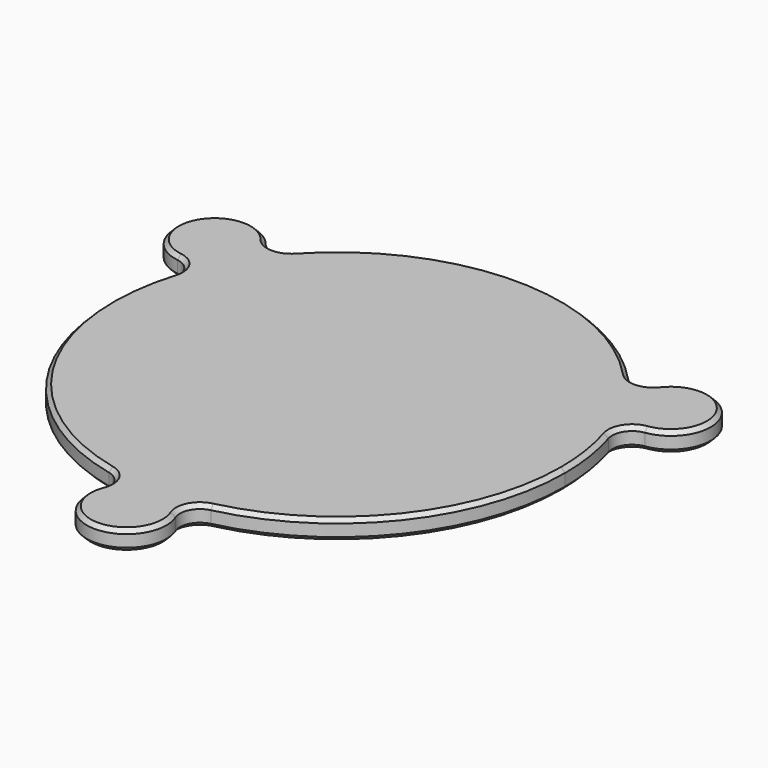
from build123d import *

# Parameters (mm, degrees)
F1_DEPTH = 5
F2_R     = 5
F3_SIZE  = 1


with BuildPart() as f1:
    # F0 (on Top) → F1 (new body)
    with BuildSketch(Plane.XY):
        with BuildLine():
            ThreePointArc((-4.0489926269, -57.0063869992), (0, -76.15), (4.0489926269, -57.0063869992))
            ThreePointArc((4.0489926269, -57.0063869992), (0, -57.15), (-4.0489926269, -57.0063869992))
        make_face()
        with BuildLine():
            ThreePointArc((4.0489926269, -57.0063869992), (41.8181923846, -38.9533218826), (57.15, 0))
            ThreePointArc((57.15, 0), (55.6922778867, 12.8254701198), (51.3934756327, 24.996663025))
            ThreePointArc((51.3934756327, 24.996663025), (49.4933518263, 28.575), (47.3444830059, 32.0097239742))
            ThreePointArc((47.3444830059, 32.0097239742), (0, 57.15), (-47.3444830059, 32.0097239742))
            ThreePointArc((-47.3444830059, 32.0097239742), (-49.4933518263, 28.575), (-51.3934756327, 24.996663025))
            ThreePointArc((-51.3934756327, 24.996663025), (-49.4933518263, -28.575), (-4.0489926269, -57.0063869992))
            ThreePointArc((-4.0489926269, -57.0063869992), (0, -57.15), (4.0489926269, -57.0063869992))
        make_face()
        with BuildLine():
            ThreePointArc((-51.3934756327, 24.996663025), (-49.4933518263, 28.575), (-47.3444830059, 32.0097239742))
            ThreePointArc((-47.3444830059, 32.0097239742), (-65.9478344982, 38.075), (-51.3934756327, 24.996663025))
        make_face()
        with BuildLine():
            ThreePointArc((47.3444830059, 32.0097239742), (49.4933518263, 28.575), (51.3934756327, 24.996663025))
            ThreePointArc((51.3934756327, 24.996663025), (65.9478344982, 38.075), (47.3444830059, 32.0097239742))
        make_face()
    extrude(amount=F1_DEPTH)

    # F2
    f2_edges = [f1.edges().sort_by_distance(p)[0] for p in [
        (-4.048993, -57.006387, 2.5),
        (51.393476, 24.996663, 2.5),
        (-47.344483, 32.009724, 2.5),
        (4.048993, -57.006387, 2.5),
        (47.344483, 32.009724, 2.5),
        (-51.393476, 24.996663, 2.5),
    ]]
    fillet(f2_edges, radius=F2_R)

    # F3
    f3_edges = [f1.edges().sort_by_distance(p)[0] for p in [
        (0, -76.15, 5),
        (-9.492901, -58.253155, 5),
        (9.492901, -58.253155, 5),
        (-49.493352, -28.575, 5),
        (49.493352, -28.575, 5),
        (-55.195163, 20.905484, 5),
        (55.195163, 20.905484, 5),
        (-65.947834, 38.075, 5),
        (65.947834, 38.075, 5),
        (-45.702262, 37.347671, 5),
        (45.702262, 37.347671, 5),
        (0, 57.15, 5),
        (0, -76.15, 0),
        (-9.492901, -58.253155, 0),
        (9.492901, -58.253155, 0),
        (-49.493352, -28.575, 0),
        (49.493352, -28.575, 0),
        (-55.195163, 20.905484, 0),
        (55.195163, 20.905484, 0),
        (-65.947834, 38.075, 0),
        (65.947834, 38.075, 0),
        (-45.702262, 37.347671, 0),
        (45.702262, 37.347671, 0),
        (0, 57.15, 0),
    ]]
    chamfer(f3_edges, length=F3_SIZE)


solid = f1.part
